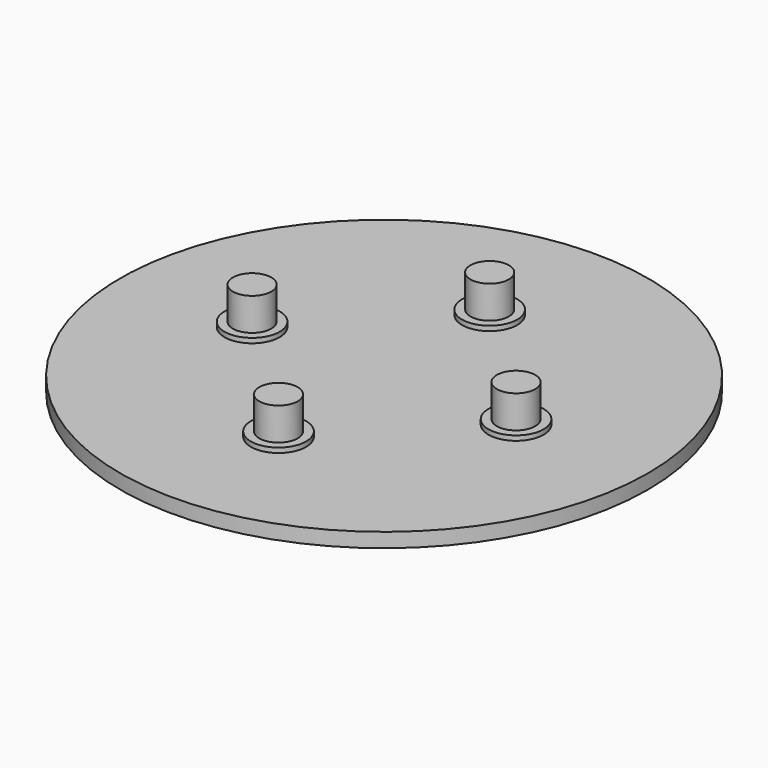
from build123d import *

# Parameters (mm, degrees)
F0_R      = 55
F1_DEPTH  = 3
F2_R      = 5.75
F3_DEPTH  = 1
F5_R      = 4
F6_DEPTH  = 6.8
F4_R      = 4
F7_DEPTH  = 6.8
F8_R      = 4
F9_DEPTH  = 6.8
F10_R     = 4
F11_DEPTH = 6.8


# Not quite as in the source:
# - a feature of the source that left no trace in its solid (it failed there, or was rolled back) is left out


with BuildPart() as f1:
    # F0 (on Top) → F1 (new body)
    with BuildSketch(Plane.XY):
        Circle(F0_R)
    extrude(amount=F1_DEPTH)

    # F2 (on face) → F3 (join)
    with BuildSketch(Plane.XY.offset(3)):
        with Locations((-27.5, 0)):
            Circle(F2_R)
        with Locations((27.5, 0)):
            Circle(F2_R)
        with Locations((0, 27.5)):
            Circle(F2_R)
        with Locations((0, -27.5)):
            Circle(F2_R)
    extrude(amount=F3_DEPTH)

    # F5 (on face) → F6 (join)
    with BuildSketch(Plane.XY.offset(4)):
        with Locations((27.5, 0)):
            Circle(F5_R)
    extrude(amount=F6_DEPTH)

    # F4 (on face) → F7 (join)
    with BuildSketch(Plane.XY.offset(4)):
        with Locations((-27.5, 0)):
            Circle(F4_R)
    extrude(amount=F7_DEPTH)

    # F8 (on face) → F9 (join)
    with BuildSketch(Plane.XY.offset(4)):
        with Locations((0, 27.5)):
            Circle(F8_R)
    extrude(amount=F9_DEPTH)

    # F10 (on face) → F11 (join)
    with BuildSketch(Plane.XY.offset(4)):
        with Locations((0, -27.5)):
            Circle(F10_R)
    extrude(amount=F11_DEPTH)


solid = f1.part
